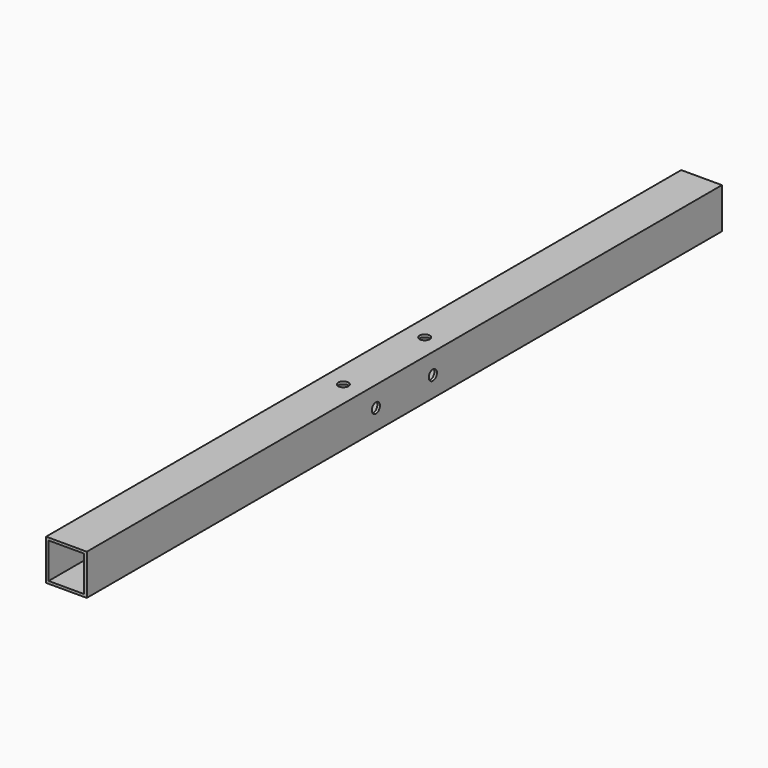
from build123d import *

# Parameters (mm, degrees)
F0_W     = 50.8
F0_H     = 50.8
F0_W_2   = 44.45
F0_H_2   = 44.45
F1_DEPTH = 495.3
F3_D     = 12.7
F3_DEPTH = 12.7
F3_TIP   = 3.8154649308
F5_D     = 12.7
F5_DEPTH = 12.7
F5_TIP   = 3.8154649308


# Not quite as in the source:
# - a length typed as a fraction of an inch, garbled in the dataset ("3 / 203.2 mm" for 3/8 in), is restored


with BuildPart() as f1:
    # F0 (on Front) → F1 (new body, symmetric)
    with BuildSketch(Plane.XZ):
        Rectangle(F0_W, F0_H)
        Rectangle(F0_W_2, F0_H_2, mode=Mode.SUBTRACT)
    extrude(amount=F1_DEPTH, both=True)

    # F3
    with Locations(Plane.XY.offset(25.4)):
        with Locations((0, 63.5), (0, -63.5)):
            Hole(F3_D / 2, depth=F3_DEPTH)
            with Locations((0, 0, -(F3_DEPTH + F3_TIP / 2))):  # 118° drill point
                Cone(0, F3_D / 2, F3_TIP, mode=Mode.SUBTRACT)

    # F5
    with Locations(Plane.YZ.offset(25.4)):
        with Locations((44.45, 0), (-44.45, 0)):
            Hole(F5_D / 2, depth=F5_DEPTH)
            with Locations((0, 0, -(F5_DEPTH + F5_TIP / 2))):  # 118° drill point
                Cone(0, F5_D / 2, F5_TIP, mode=Mode.SUBTRACT)


solid = f1.part
